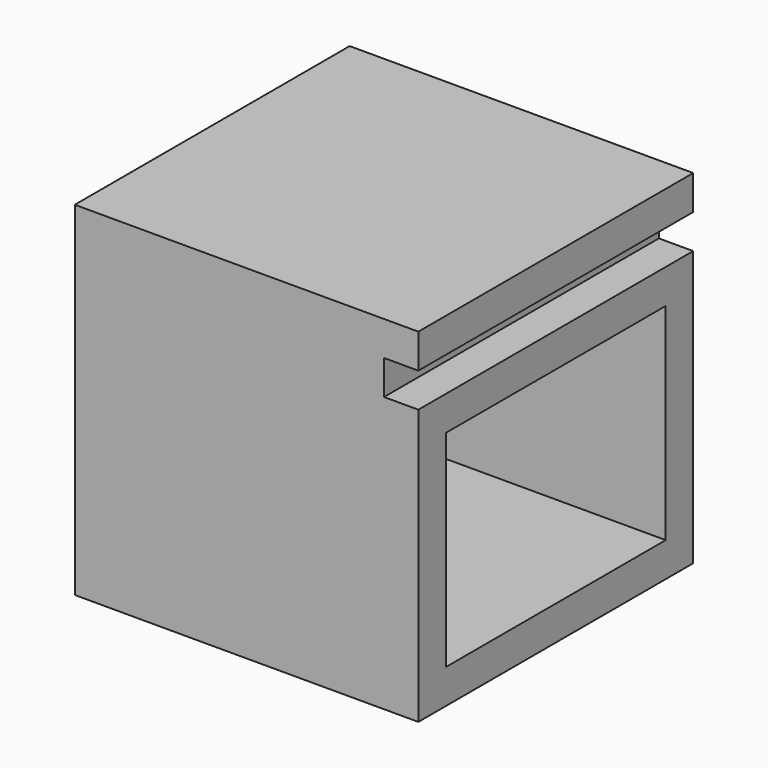
from build123d import *

# Parameters (mm, degrees)
F1_DEPTH = 25.4
F2_T     = -2.54


with BuildPart() as f1:
    # F0 (on Front) → F1 (new body)
    with BuildSketch(Plane.XZ):
        Polygon((0, 25.4), (0, 0), (25.4, 0), (25.4, 20.32), (22.86, 20.32), (22.86, 22.86), (25.4, 22.86), (25.4, 25.4), align=None)
    extrude(amount=F1_DEPTH)

    # F2
    f2_openings = [f1.faces().sort_by_distance(p)[0] for p in [
        (25.4, -12.7, 10.16),
    ]]
    offset(amount=F2_T, openings=f2_openings, kind=Kind.INTERSECTION)


solid = f1.part
